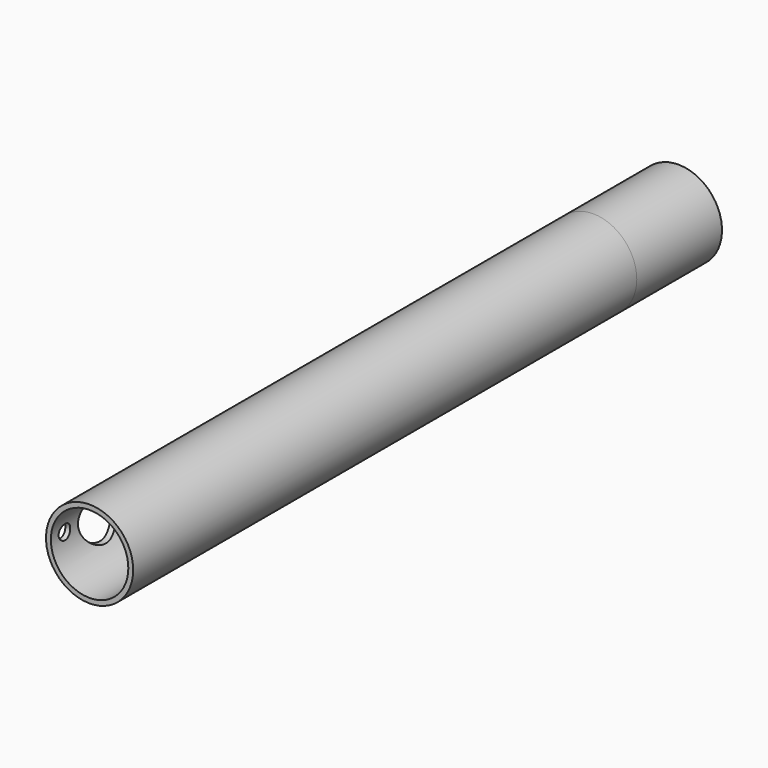
from build123d import *

# Parameters (mm, degrees)
F3_R      = 4.5
F4_DEPTH  = 42.5
F8_DEPTH  = 42.5
F6_R      = 4.5
F6_R_2    = 4
F9_DEPTH  = 22.5
F7_R      = 4.5
F7_R_2    = 4
F10_DEPTH = 11
F11_R     = 2.5
F11_R_2   = 0.75
F12_DEPTH = 4.501


# Not quite as in the source:
# - ends of sketch curves that miss each other by under 0.0002 mm in the source are joined


with BuildPart() as f4:
    # F3 (on Front) → F4 (new body)
    with BuildSketch(Plane.XZ):
        Circle(F3_R)
    extrude(amount=F4_DEPTH)

    # F5 (on face) → F8 (cut, through all)
    with BuildSketch(Plane.XZ.offset(42.5)):
        with BuildLine():
            Line((-1.25, -3.8), (0, -3.8))
            Line((0, -3.8), (1.25, -3.8))
            Line((1.25, -3.8), (1.25, -3.7))
            ThreePointArc((1.25, -3.7), (1.3085786438, -3.5585786438), (1.45, -3.5))
            Line((1.45, -3.5), (2, -3.5))
            Line((2, -3.5), (2, -3.05))
            ThreePointArc((2, -3.05), (2.0585786438, -2.9085786438), (2.2, -2.85))
            Line((2.2, -2.85), (3.15, -2.85))
            Line((3.15, -2.85), (3.15, -2.15))
            Line((3.15, -2.15), (2.2, -2.15))
            ThreePointArc((2.2, -2.15), (2.0585786438, -2.0914213562), (2, -1.95))
            Line((2, -1.95), (2, -1.887459))
            ThreePointArc((2, -1.887459), (2.1033535752, -1.771554046), (2.2, -1.65))
            Line((2.2, -1.65), (3.75, -1.65))
            Line((3.75, -1.65), (3.75, 0))
            Line((3.75, 0), (3.75, 1.65))
            Line((3.75, 1.65), (2.2, 1.65))
            ThreePointArc((2.2, 1.65), (2.1033535752, 1.771554046), (1.9999998047, 1.8874588157))
            Line((1.9999998047, 1.8874588157), (2, 1.95))
            ThreePointArc((2, 1.95), (2.0585786438, 2.0914213562), (2.2, 2.15))
            Line((2.2, 2.15), (3.15, 2.15))
            Line((3.15, 2.15), (3.15, 2.85))
            Line((3.15, 2.85), (2.2, 2.85))
            ThreePointArc((2.2, 2.85), (2.0585786438, 2.9085786438), (2, 3.05))
            Line((2, 3.05), (2, 3.5))
            Line((2, 3.5), (1.45, 3.5))
            ThreePointArc((1.45, 3.5), (1.3085786438, 3.5585786438), (1.25, 3.7))
            Line((1.25, 3.7), (1.25, 3.8))
            Line((1.25, 3.8), (0, 3.8))
            Line((0, 3.8), (-1.25, 3.8))
            Line((-1.25, 3.8), (-1.25, 3.7))
            ThreePointArc((-1.25, 3.7), (-1.3085786438, 3.5585786438), (-1.45, 3.5))
            Line((-1.45, 3.5), (-2, 3.5))
            Line((-2, 3.5), (-2, 3.05))
            ThreePointArc((-2, 3.05), (-2.0585786438, 2.9085786438), (-2.2, 2.85))
            Line((-2.2, 2.85), (-3.15, 2.85))
            Line((-3.15, 2.85), (-3.15, 2.15))
            Line((-3.15, 2.15), (-2.2, 2.15))
            ThreePointArc((-2.2, 2.15), (-2.0585786438, 2.0914213562), (-2, 1.95))
            Line((-2, 1.95), (-2, 1.887459))
            ThreePointArc((-2, 1.887459), (-2.1033535752, 1.771554046), (-2.2, 1.65))
            Line((-2.2, 1.65), (-3.75, 1.65))
            Line((-3.75, 1.65), (-3.75, 0))
            Line((-3.75, 0), (-3.75, -1.65))
            Line((-3.75, -1.65), (-2.2, -1.65))
            ThreePointArc((-2.2, -1.65), (-2.1033535752, -1.771554046), (-1.9999998047, -1.8874588157))
            Line((-1.9999998047, -1.8874588157), (-2, -1.95))
            ThreePointArc((-2, -1.95), (-2.0585786438, -2.0914213562), (-2.2, -2.15))
            Line((-2.2, -2.15), (-3.15, -2.15))
            Line((-3.15, -2.15), (-3.15, -2.85))
            Line((-3.15, -2.85), (-2.2, -2.85))
            ThreePointArc((-2.2, -2.85), (-2.0585786438, -2.9085786438), (-2, -3.05))
            Line((-2, -3.05), (-2, -3.5))
            Line((-2, -3.5), (-1.45, -3.5))
            ThreePointArc((-1.45, -3.5), (-1.3085786438, -3.5585786438), (-1.25, -3.7))
            Line((-1.25, -3.7), (-1.25, -3.8))
        make_face()
    extrude(amount=-F8_DEPTH, mode=Mode.SUBTRACT)

    # F6 (on face) → F9 (join)
    with BuildSketch(Plane.XZ.offset(42.5)):
        Circle(F6_R)
        Circle(F6_R_2, mode=Mode.SUBTRACT)
    extrude(amount=F9_DEPTH)

    # F7 (on face) → F10 (join)
    with BuildSketch(Plane(origin=(0, 0, 0), x_dir=(-1, 0, 0), z_dir=(0, 1, 0))):
        Circle(F7_R)
        Circle(F7_R_2, mode=Mode.SUBTRACT)
    extrude(amount=F10_DEPTH)

    # F11 (on Right) → F12 (cut, through all)
    with BuildSketch(Plane.YZ):
        with Locations((-59, 0)):
            Circle(F11_R)
        with Locations((-63.25, 0)):
            Circle(F11_R_2)
    extrude(amount=-F12_DEPTH, mode=Mode.SUBTRACT)


solid = f4.part
